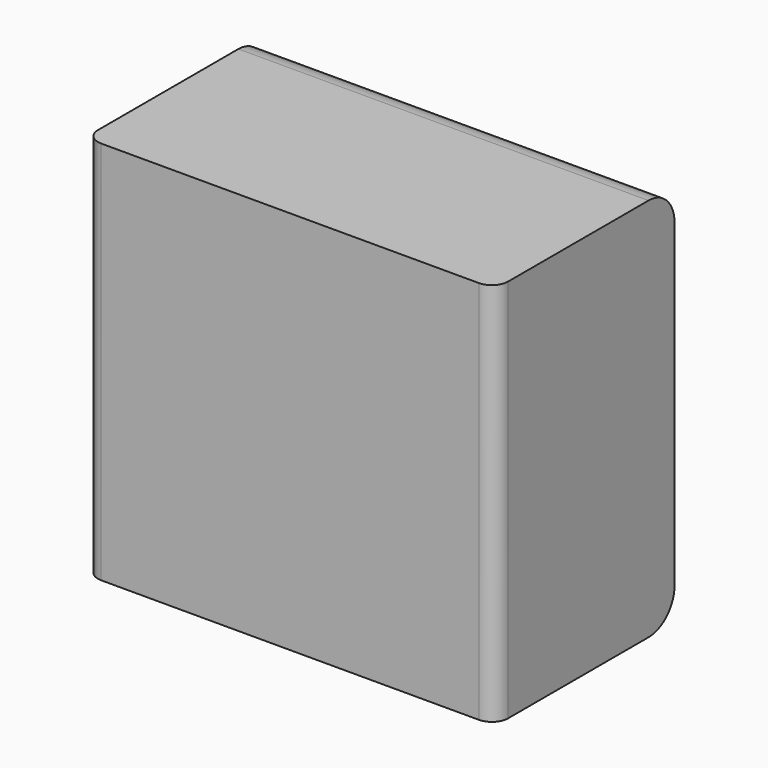
from build123d import *

# Parameters (mm, degrees)
F0_W        = 64
F0_H        = 60
F1_DEPTH    = 35
F2_T        = -2
F3_R        = 5.08
F4_T1_DEPTH = 89.4
F5_R        = 2.54


# Not quite as in the source:
# - a fillet or chamfer that OpenCascade refuses, or shapes differently, is made with other operations: its cross-section is extruded or revolved along the edge and cut away or added


with BuildPart() as f1:
    # F0 (on Front) → F1 (new body)
    with BuildSketch(Plane.XZ):
        with Locations((-1.7414748222, 19.6752779907)):
            Rectangle(F0_W, F0_H)
    extrude(amount=F1_DEPTH)

    # F2
    f2_openings = [f1.faces().sort_by_distance(p)[0] for p in [
        (-1.741475, -17.5, -10.324722),
    ]]
    offset(amount=F2_T, openings=f2_openings)

    # F3
    f3_edges = [f1.edges().sort_by_distance(p)[0] for p in [
        (-1.741475, 0, 49.675278),
    ]]
    fillet(f3_edges, radius=F3_R)

    # F4: fillet of radius 5.08 on 1 edges, made by hand

    # F4_s2 → F4_t1 (cut)
    with BuildSketch(Plane.YZ.offset(-46.4414748222)):
        with BuildLine():
            ThreePointArc((0, -5.2447220093), (-1.4878975516, -8.8368244577), (-5.08, -10.3247220093))
            Line((-5.08, -10.3247220093), (0, -10.3247220093))
            Line((0, -10.3247220093), (0, -5.2447220093))
        make_face()
    extrude(amount=F4_T1_DEPTH, mode=Mode.SUBTRACT)

    # F5
    f5_edges = [f1.edges().sort_by_distance(p)[0] for p in [
        (-33.741475, -35, 19.675278),
        (30.258525, -35, 19.675278),
    ]]
    fillet(f5_edges, radius=F5_R)


solid = f1.part
